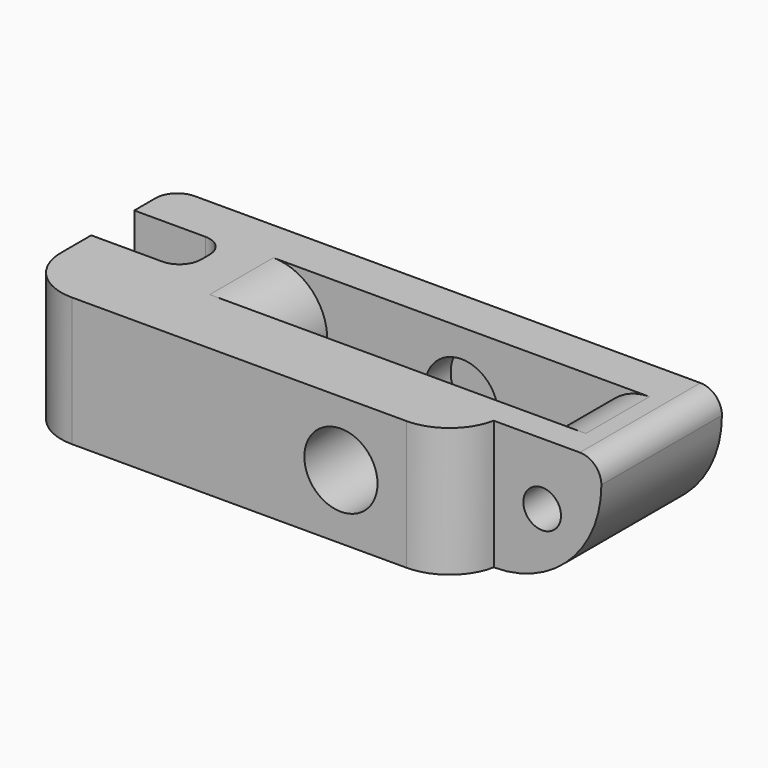
from build123d import *

# Parameters (mm, degrees)
F0_W        = 41
F0_H        = 4
F1_DEPTH    = 6
F3_START    = -6.6
F2_R        = 3.4
F3_DEPTH    = 7.4
F4_T1_DEPTH = 37
F4_T3_DEPTH = 36.4948974279
F4_T5_DEPTH = 7.4
F4_T7_DEPTH = 7.4
F5_DEPTH    = 17
F6_R        = 10
F7_R        = 1.99999
F8_R        = 2
F2_R_2      = 1.75
F9_DEPTH    = 18.001


# Not quite as in the source:
# - a fillet or chamfer that OpenCascade refuses, or shapes differently, is made with other operations: its cross-section is extruded or revolved along the edge and cut away or added
# - a fillet or chamfer is up to 0.001 mm smaller than in the source, because OpenCascade refuses the exact size


with BuildPart() as f1:
    # F0 (on Top) → F1 (new body, symmetric)
    with BuildSketch(Plane.XY):
        Polygon((11, -4.5), (21, -4.5), (21, 9.5), (-30, 9.5), (-30, 5), (-21.4, 5), (-21.4, 0), (-30, 0), (-30, -4.5), align=None)
        with Locations((-9.5, -6.5)):
            Rectangle(F0_W, F0_H)
    extrude(amount=F1_DEPTH, both=True)

    # F2 (on face) → F3 (cut)
    with BuildSketch(Plane.XZ.offset(8.5).offset(F3_START)):
        with BuildLine():
            Line((11, -5.9371710435), (11, 5.9371710435))
            ThreePointArc((11, 5.9371710435), (10.9829729772, 5.9686099372), (10.9658560997, 6))
            Line((10.9658560997, 6), (-10.9658560997, 6))
            ThreePointArc((-10.9658560997, 6), (-12.5, 0), (-10.9658560997, -6))
            Line((-10.9658560997, -6), (10.9658560997, -6))
            ThreePointArc((10.9658560997, -6), (10.9829729772, -5.9686099372), (11, -5.9371710435))
        make_face()
        Circle(F2_R, mode=Mode.SUBTRACT)
        with BuildLine():
            ThreePointArc((11, -5.9371710435), (12.1191996435, -3.0618621785), (12.5, 0))
            ThreePointArc((12.5, 0), (12.1191996435, 3.0618621785), (11, 5.9371710435))
            Line((11, 5.9371710435), (11, -5.9371710435))
        make_face()
        Circle(F2_R)
    extrude(amount=-F3_DEPTH, mode=Mode.SUBTRACT)

    # F4: fillet of radius 5 on 4 edges, made by hand

    # F4_s2 → F4_t1 (cut)
    with BuildSketch(Plane.XY.offset(-18.5)):
        with BuildLine():
            ThreePointArc((-25, -8.5), (-28.5355339059, -7.0355339059), (-30, -3.5))
            Line((-30, -3.5), (-30, -8.5))
            Line((-30, -8.5), (-25, -8.5))
        make_face()
    extrude(amount=F4_T1_DEPTH, mode=Mode.SUBTRACT)

    # F4_s4 → F4_t3 (cut)
    with BuildSketch(Plane.XY.offset(-18.2474487139)):
        with BuildLine():
            ThreePointArc((11, -4.5), (9.2632981746, -7.3729833462), (6.1010205144, -8.5))
            Line((6.1010205144, -8.5), (11, -8.5))
            Line((11, -8.5), (11, -4.5))
        make_face()
    extrude(amount=F4_T3_DEPTH, mode=Mode.SUBTRACT)

    # F4_s6 → F4_t5 (cut)
    with BuildSketch(Plane.XZ.offset(-5.5)):
        with BuildLine():
            ThreePointArc((-17.4714052097, 6), (-13.8362593097, 4.4330328116), (-12.4795751498, 0.7142857143))
            ThreePointArc((-12.4795751498, 0.7142857143), (-12.0169361942, 3.4414015319), (-10.9658560997, 6))
            Line((-10.9658560997, 6), (-17.4714052097, 6))
        make_face()
    extrude(amount=F4_T5_DEPTH, mode=Mode.SUBTRACT)

    # F4_s8 → F4_t7 (cut)
    with BuildSketch(Plane.XZ.offset(-5.5)):
        with BuildLine():
            ThreePointArc((17.4714052097, 6), (13.8362593097, 4.4330328116), (12.4795751498, 0.7142857143))
            ThreePointArc((12.4795751498, 0.7142857143), (12.0169361943, 3.4414015319), (10.9658560997, 6))
            Line((10.9658560997, 6), (17.4714052097, 6))
        make_face()
    extrude(amount=F4_T7_DEPTH, mode=Mode.SUBTRACT)

    # F2 (on face) → F5 (cut, through all)
    with BuildSketch(Plane.XZ.offset(8.5)):
        Circle(F2_R)
    extrude(amount=-F5_DEPTH, mode=Mode.SUBTRACT)

    # F6
    f6_edges = [f1.edges().sort_by_distance(p)[0] for p in [
        (21, 2.5, -6),
    ]]
    fillet(f6_edges, radius=F6_R)

    # F7 (radius 2 in the source; OpenCascade refuses exactly that, so slightly less here)
    f7_edges = [f1.edges().sort_by_distance(p)[0] for p in [
        (21, 2.5, 6),
    ]]
    fillet(f7_edges, radius=F7_R)

    # F8
    f8_edges = [f1.edges().sort_by_distance(p)[0] for p in [
        (-30, 9.5, 0),
        (-21.4, 5, 0),
        (-21.4, 0, 0),
    ]]
    fillet(f8_edges, radius=F8_R)

    # F2 (on face) → F9 (cut, through all)
    with BuildSketch(Plane.XZ.offset(8.5)):
        with Locations((15.5, 0.25)):
            Circle(F2_R_2)
    extrude(amount=-F9_DEPTH, mode=Mode.SUBTRACT)


solid = f1.part
